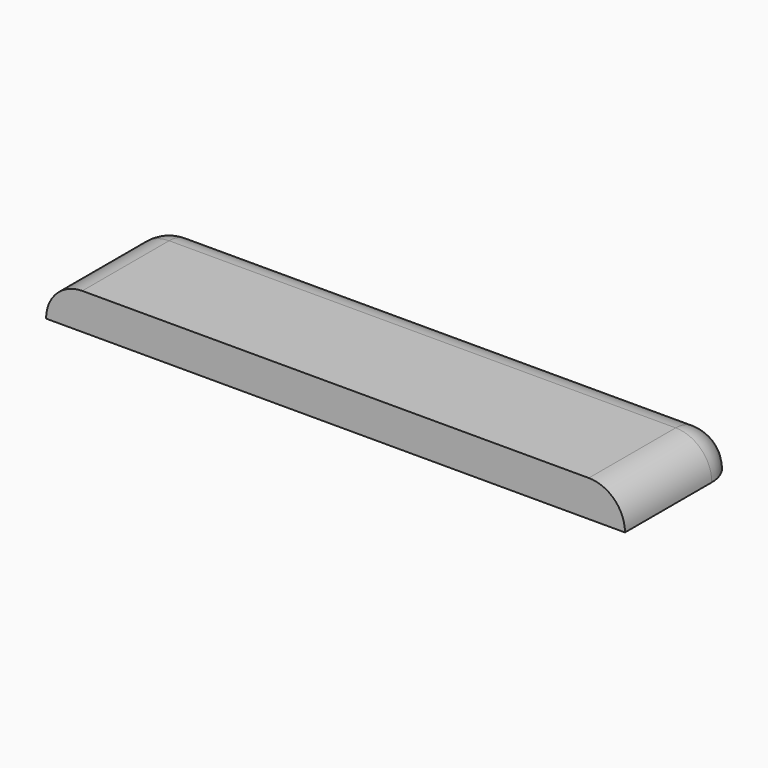
from build123d import *

# Parameters (mm, degrees)
F1_DEPTH = 6.35
F2_R     = 6.34999


# Not quite as in the source:
# - a fillet or chamfer is up to 0.001 mm smaller than in the source, because OpenCascade refuses the exact size


with BuildPart() as f1:
    # F0 (on Top) → F1 (new body)
    with BuildSketch(Plane.XY):
        with BuildLine():
            ThreePointArc((50.8, 6.35), (48.9401280605, 10.8401280605), (44.45, 12.7))
            Line((44.45, 12.7), (-44.45, 12.7))
            ThreePointArc((-44.45, 12.7), (-48.9401280605, 10.8401280605), (-50.8, 6.35))
            Line((-50.8, 6.35), (-50.8, -12.7))
            Line((-50.8, -12.7), (50.8, -12.7))
            Line((50.8, -12.7), (50.8, 6.35))
        make_face()
    extrude(amount=F1_DEPTH)

    # F2 (radius 6.35 in the source; OpenCascade refuses exactly that, so slightly less here)
    f2_edges = [f1.edges().sort_by_distance(p)[0] for p in [
        (0, 12.7, 6.35),
    ]]
    fillet(f2_edges, radius=F2_R)


solid = f1.part
